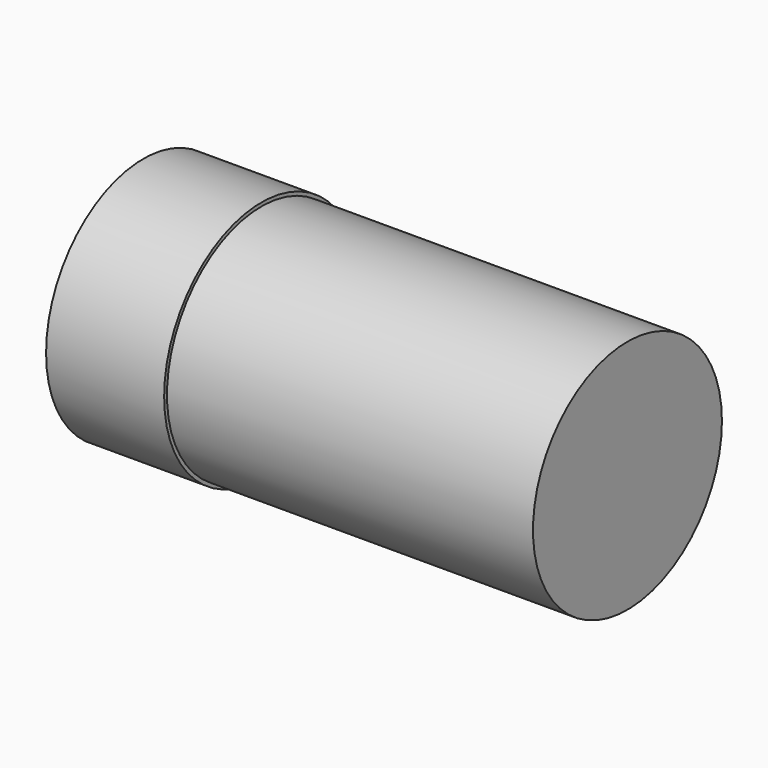
from build123d import *

# Parameters (mm, degrees)
F0_R     = 51.5
F0_R_2   = 50
F1_DEPTH = 45
F2_DEPTH = 200
F3_DEPTH = 5
F4_T     = 2.5


# Not quite as in the source:
# - a shell that OpenCascade refuses in one call is made with other operations: the cavity is built on its own and cut out


with BuildPart() as f1:
    # F0 (on Right) → F1 (new body)
    with BuildSketch(Plane.YZ):
        Circle(F0_R)
        Circle(F0_R_2, mode=Mode.SUBTRACT)
    extrude(amount=F1_DEPTH)

    # F0 (on Right) → F2 (join)
    with BuildSketch(Plane.YZ):
        Circle(F0_R_2)
    extrude(amount=F2_DEPTH)

    # F0 (on Right) → F3 (join)
    with BuildSketch(Plane.YZ):
        Circle(F0_R)
        Circle(F0_R_2, mode=Mode.SUBTRACT)
    extrude(amount=-F3_DEPTH)

    # F4: shell of thickness 2.5, made by hand


with BuildPart() as f4_core1:
    # F4_t2: copy of F1
    add(f1.part)

    # the walls: a layer under each face that stays
    f4_faces = [f4_core1.faces().sort_by_distance(p)[0] for p in [
        (22.5, -51.5, 0),
        (-2.5, -51.5, 0),
        (45, 45.0625, -24.7962962963),
        (-5, 45.0625, -24.7962962963),
        (122.5, -50, 0),
        (-2.5, -50, 0),
        (200, 0, 0),
    ]]
    thicken(f4_faces, amount=-F4_T, mode=Mode.SUBTRACT)

    # F4_s3 → F4_t4 (revolve, cut)
    with BuildSketch(Plane.XY):
        Polygon((45.025, 50.025), (42.5, 50), (42.5, 47.5), (45, 47.5), align=None)
    revolve(axis=Axis((45, 0, 0), (1, 0, 0)), mode=Mode.SUBTRACT)


with BuildPart() as f1_1:
    add(f1.part)

    # what is left inside the walls is the cavity
    f4_cavity = [f4_core1.part.solids().sort_by_distance(p)[0] for p in [
        (146.666667, -47.475, 0),
    ]]
    add(f4_cavity, mode=Mode.SUBTRACT)


solid = f1_1.part
